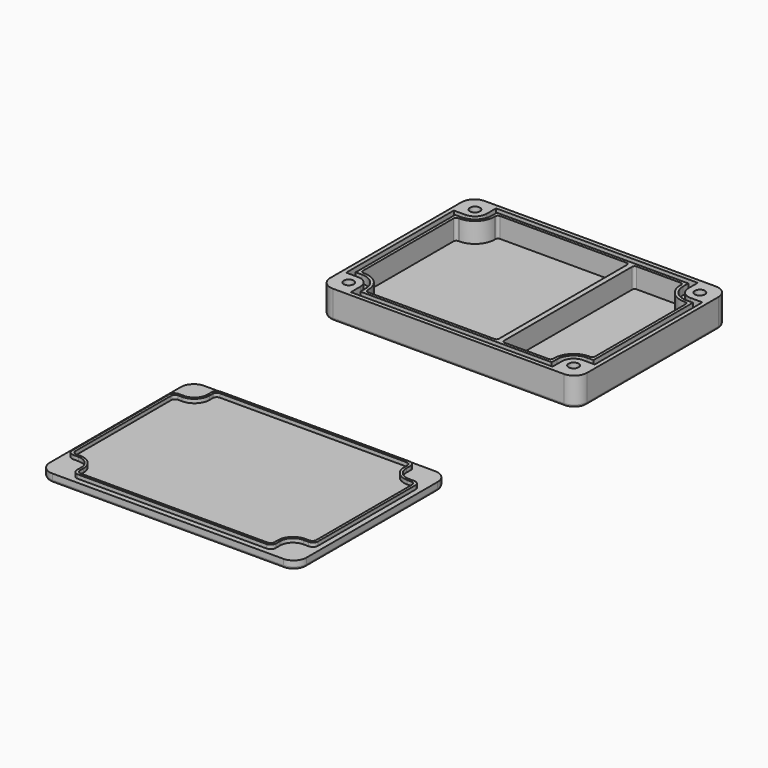
from build123d import *

# Parameters (mm, degrees)
F0_R      = 1.95
F1_DEPTH  = 11
F2_DEPTH  = 8
F3_DEPTH  = 3.2
F4_R      = 1.25
F5_DEPTH  = 3.2
F4_W      = 2
F4_H      = 66.4
F6_DEPTH  = 4.7
F4_R_2    = 2.75
F7_DEPTH  = 3.2
F8_DEPTH  = 3.2
F9_DEPTH  = 3.2
F10_R     = 1
F10_2_R   = 1
F12_R     = 3.65
F12_R_2   = 1.95
F13_DEPTH = 3.7
F17_DEPTH = 1.5
F18_DEPTH = 1.5
F19_R     = 2


# Not quite as in the source:
# - two fillets or chamfers of one size are made in one step


with BuildPart() as f1:
    # F0 (on Top) → F1 (new body)
    with BuildSketch(Plane.XY):
        with BuildLine():
            Line((56.8, 36.8), (-32.8, 36.8))
            ThreePointArc((-32.8, 36.8), (-36.3355339059, 35.3355339059), (-37.8, 31.8))
            Line((-37.8, 31.8), (-37.8, -31.8))
            ThreePointArc((-37.8, -31.8), (-36.3355339059, -35.3355339059), (-32.8, -36.8))
            Line((-32.8, -36.8), (56.8, -36.8))
            ThreePointArc((56.8, -36.8), (60.3355339059, -35.3355339059), (61.8, -31.8))
            Line((61.8, -31.8), (61.8, 31.8))
            ThreePointArc((61.8, 31.8), (60.3355339059, 35.3355339059), (56.8, 36.8))
        make_face()
        with Locations((-31.6, -30.6)):
            Circle(F0_R, mode=Mode.SUBTRACT)
        with Locations((55.6, -30.6)):
            Circle(F0_R, mode=Mode.SUBTRACT)
        with BuildLine():
            Line((51.1, -35.2), (-27.1, -35.2))
            Line((-27.1, -35.2), (-27.1, -30.6))
            ThreePointArc((-27.1, -30.6), (-28.4180194847, -27.4180194847), (-31.6, -26.1))
            Line((-31.6, -26.1), (-36.2, -26.1))
            Line((-36.2, -26.1), (-36.2, 26.1))
            Line((-36.2, 26.1), (-31.6, 26.1))
            ThreePointArc((-31.6, 26.1), (-28.4180194847, 27.4180194847), (-27.1, 30.6))
            Line((-27.1, 30.6), (-27.1, 35.2))
            Line((-27.1, 35.2), (51.1, 35.2))
            Line((51.1, 35.2), (51.1, 30.6))
            ThreePointArc((51.1, 30.6), (52.4180194847, 27.4180194847), (55.6, 26.1))
            Line((55.6, 26.1), (60.2, 26.1))
            Line((60.2, 26.1), (60.2, -26.1))
            Line((60.2, -26.1), (55.6, -26.1))
            ThreePointArc((55.6, -26.1), (52.4180194847, -27.4180194847), (51.1, -30.6))
            Line((51.1, -30.6), (51.1, -35.2))
        make_face(mode=Mode.SUBTRACT)
        with Locations((-31.6, 30.6)):
            Circle(F0_R, mode=Mode.SUBTRACT)
        with Locations((55.6, 30.6)):
            Circle(F0_R, mode=Mode.SUBTRACT)
    extrude(amount=F1_DEPTH)



with BuildPart() as f1b:
    # F0 (on Top) → F1, piece 2 (new body)
    with BuildSketch(Plane.XY):
        with BuildLine():
            Line((49.1, 33.1), (-25.1, 33.1))
            Line((-25.1, 33.1), (-25.1, 30.6))
            ThreePointArc((-25.1, 30.6), (-27.0038059223, 26.0038059223), (-31.6, 24.1))
            Line((-31.6, 24.1), (-34.1, 24.1))
            Line((-34.1, 24.1), (-34.1, -24.1))
            Line((-34.1, -24.1), (-31.6, -24.1))
            ThreePointArc((-31.6, -24.1), (-27.0038059223, -26.0038059223), (-25.1, -30.6))
            Line((-25.1, -30.6), (-25.1, -33.1))
            Line((-25.1, -33.1), (49.1, -33.1))
            Line((49.1, -33.1), (49.1, -30.6))
            ThreePointArc((49.1, -30.6), (51.0038059223, -26.0038059223), (55.6, -24.1))
            Line((55.6, -24.1), (58.1, -24.1))
            Line((58.1, -24.1), (58.1, 24.1))
            Line((58.1, 24.1), (55.6, 24.1))
            ThreePointArc((55.6, 24.1), (51.0038059223, 26.0038059223), (49.1, 30.6))
            Line((49.1, 30.6), (49.1, 33.1))
        make_face()
        with BuildLine():
            Line((-24, 30.6), (-24, 32))
            Line((-24, 32), (27, 32))
            Line((27, 32), (27, -32))
            Line((27, -32), (-24, -32))
            Line((-24, -32), (-24, -30.6))
            ThreePointArc((-24, -30.6), (-26.225988463, -25.225988463), (-31.6, -23))
            Line((-31.6, -23), (-33, -23))
            Line((-33, -23), (-33, 23))
            Line((-33, 23), (-31.6, 23))
            ThreePointArc((-31.6, 23), (-26.225988463, 25.225988463), (-24, 30.6))
        make_face(mode=Mode.SUBTRACT)
        with BuildLine():
            Line((55.6, 23), (57, 23))
            Line((57, 23), (57, -23))
            Line((57, -23), (55.6, -23))
            ThreePointArc((55.6, -23), (50.225988463, -25.225988463), (48, -30.6))
            Line((48, -30.6), (48, -32))
            Line((48, -32), (29, -32))
            Line((29, -32), (29, 32))
            Line((29, 32), (48, 32))
            Line((48, 32), (48, 30.6))
            ThreePointArc((48, 30.6), (50.225988463, 25.225988463), (55.6, 23))
        make_face(mode=Mode.SUBTRACT)
    extrude(amount=F1_DEPTH)


with BuildPart() as f1_1:
    add(f1.part)

    add(f1b.part)  # F2 merges F1b
    # F0 (on Top) → F2 (join)
    with BuildSketch(Plane.XY):
        with BuildLine():
            Line((-27.1, -30.6), (-27.1, -35.2))
            Line((-27.1, -35.2), (51.1, -35.2))
            Line((51.1, -35.2), (51.1, -30.6))
            ThreePointArc((51.1, -30.6), (52.4180194847, -27.4180194847), (55.6, -26.1))
            Line((55.6, -26.1), (60.2, -26.1))
            Line((60.2, -26.1), (60.2, 26.1))
            Line((60.2, 26.1), (55.6, 26.1))
            ThreePointArc((55.6, 26.1), (52.4180194847, 27.4180194847), (51.1, 30.6))
            Line((51.1, 30.6), (51.1, 35.2))
            Line((51.1, 35.2), (-27.1, 35.2))
            Line((-27.1, 35.2), (-27.1, 30.6))
            ThreePointArc((-27.1, 30.6), (-28.4180194847, 27.4180194847), (-31.6, 26.1))
            Line((-31.6, 26.1), (-36.2, 26.1))
            Line((-36.2, 26.1), (-36.2, -26.1))
            Line((-36.2, -26.1), (-31.6, -26.1))
            ThreePointArc((-31.6, -26.1), (-28.4180194847, -27.4180194847), (-27.1, -30.6))
        make_face()
        with BuildLine():
            Line((-25.1, 30.6), (-25.1, 33.1))
            Line((-25.1, 33.1), (49.1, 33.1))
            Line((49.1, 33.1), (49.1, 30.6))
            ThreePointArc((49.1, 30.6), (51.0038059223, 26.0038059223), (55.6, 24.1))
            Line((55.6, 24.1), (58.1, 24.1))
            Line((58.1, 24.1), (58.1, -24.1))
            Line((58.1, -24.1), (55.6, -24.1))
            ThreePointArc((55.6, -24.1), (51.0038059223, -26.0038059223), (49.1, -30.6))
            Line((49.1, -30.6), (49.1, -33.1))
            Line((49.1, -33.1), (-25.1, -33.1))
            Line((-25.1, -33.1), (-25.1, -30.6))
            ThreePointArc((-25.1, -30.6), (-27.0038059223, -26.0038059223), (-31.6, -24.1))
            Line((-31.6, -24.1), (-34.1, -24.1))
            Line((-34.1, -24.1), (-34.1, 24.1))
            Line((-34.1, 24.1), (-31.6, 24.1))
            ThreePointArc((-31.6, 24.1), (-27.0038059223, 26.0038059223), (-25.1, 30.6))
        make_face(mode=Mode.SUBTRACT)
    extrude(amount=F2_DEPTH)

    # F0 (on Top) → F3 (join)
    with BuildSketch(Plane.XY):
        with BuildLine():
            Line((57, -23), (57, 23))
            Line((57, 23), (55.6, 23))
            ThreePointArc((55.6, 23), (50.225988463, 25.225988463), (48, 30.6))
            Line((48, 30.6), (48, 32))
            Line((48, 32), (29, 32))
            Line((29, 32), (29, -32))
            Line((29, -32), (48, -32))
            Line((48, -32), (48, -30.6))
            ThreePointArc((48, -30.6), (50.225988463, -25.225988463), (55.6, -23))
            Line((55.6, -23), (57, -23))
        make_face()
        with BuildLine():
            Line((27, 32), (-24, 32))
            Line((-24, 32), (-24, 30.6))
            ThreePointArc((-24, 30.6), (-26.225988463, 25.225988463), (-31.6, 23))
            Line((-31.6, 23), (-33, 23))
            Line((-33, 23), (-33, -23))
            Line((-33, -23), (-31.6, -23))
            ThreePointArc((-31.6, -23), (-26.225988463, -25.225988463), (-24, -30.6))
            Line((-24, -30.6), (-24, -32))
            Line((-24, -32), (27, -32))
            Line((27, -32), (27, 32))
        make_face()
    extrude(amount=F3_DEPTH)

    # F10#2
    f10_2_edges = [f1_1.edges().sort_by_distance(p)[0] for p in [
        (-24, 32, 7.1),
        (27, 32, 7.1),
        (27, -32, 7.1),
        (-24, -32, 7.1),
        (-33, -23, 7.1),
        (-33, 23, 7.1),
        (57, 23, 7.1),
        (57, -23, 7.1),
        (48, -32, 7.1),
        (29, -32, 7.1),
        (29, 32, 7.1),
        (48, 32, 7.1),
        (12, 36.8, 0),
        (-36.335534, 35.335534, 0),
        (-37.8, 0, 0),
        (-36.335534, -35.335534, 0),
        (12, -36.8, 0),
        (60.335534, -35.335534, 0),
        (61.8, 0, 0),
        (60.335534, 35.335534, 0),
    ]]
    fillet(f10_2_edges, radius=F10_2_R)

    # F12 (on face) → F13 (cut)
    with BuildSketch(Plane(origin=(0, 0, 0), x_dir=(1, 0, 0), z_dir=(0, 0, -1))):
        with Locations((55.6, -30.6)):
            Circle(F12_R)
        with Locations((55.6, -30.6)):
            Circle(F12_R_2, mode=Mode.SUBTRACT)
        with Locations((55.6, 30.6)):
            Circle(F12_R)
        with Locations((55.6, 30.6)):
            Circle(F12_R_2, mode=Mode.SUBTRACT)
        with Locations((-31.6, -30.6)):
            Circle(F12_R)
        with Locations((-31.6, -30.6)):
            Circle(F12_R_2, mode=Mode.SUBTRACT)
        with Locations((-31.6, 30.6)):
            Circle(F12_R)
        with Locations((-31.6, 30.6)):
            Circle(F12_R_2, mode=Mode.SUBTRACT)
    extrude(amount=-F13_DEPTH, mode=Mode.SUBTRACT)


with BuildPart() as f5:
    # F4 (on Top) → F5 (new body)
    with BuildSketch(Plane.XY):
        with BuildLine():
            Line((56.8, -99.2), (-32.8, -99.2))
            ThreePointArc((-32.8, -99.2), (-36.3355339059, -100.6644660941), (-37.8, -104.2))
            Line((-37.8, -104.2), (-37.8, -167.8))
            ThreePointArc((-37.8, -167.8), (-36.3355339059, -171.3355339059), (-32.8, -172.8))
            Line((-32.8, -172.8), (56.8, -172.8))
            ThreePointArc((56.8, -172.8), (60.3355339059, -171.3355339059), (61.8, -167.8))
            Line((61.8, -167.8), (61.8, -104.2))
            ThreePointArc((61.8, -104.2), (60.3355339059, -100.6644660941), (56.8, -99.2))
        make_face()
        with Locations((-31.6, -166.6)):
            Circle(F4_R, mode=Mode.SUBTRACT)
        with Locations((55.6, -166.6)):
            Circle(F4_R, mode=Mode.SUBTRACT)
        with BuildLine():
            Line((-27, -105.4), (-27, -100.9))
            Line((-27, -100.9), (51, -100.9))
            Line((51, -100.9), (51.0491758988, -100.9))
            ThreePointArc((51.0491758988, -100.9), (51.0245188805, -100.9250729028), (51, -100.9502809077))
            Line((51, -100.9502809077), (51, -105.4))
            ThreePointArc((51, -105.4), (52.3473088065, -108.6526911935), (55.6, -110))
            Line((55.6, -110), (60.0497190923, -110))
            ThreePointArc((60.0497190923, -110), (60.0749270972, -109.9754811195), (60.1, -109.9508241012))
            Line((60.1, -109.9508241012), (60.1, -110))
            Line((60.1, -110), (60.1, -162))
            Line((60.1, -162), (60.1, -162.0491758988))
            ThreePointArc((60.1, -162.0491758988), (60.0749270972, -162.0245188805), (60.0497190923, -162))
            Line((60.0497190923, -162), (55.6, -162))
            ThreePointArc((55.6, -162), (52.3473088065, -163.3473088065), (51, -166.6))
            Line((51, -166.6), (51, -171.0497190923))
            ThreePointArc((51, -171.0497190923), (51.0245188805, -171.0749270972), (51.0491758988, -171.1))
            Line((51.0491758988, -171.1), (51, -171.1))
            Line((51, -171.1), (-27, -171.1))
            Line((-27, -171.1), (-27.0491758988, -171.1))
            ThreePointArc((-27.0491758988, -171.1), (-27.0245188805, -171.0749270972), (-27, -171.0497190923))
            Line((-27, -171.0497190923), (-27, -166.6))
            ThreePointArc((-27, -166.6), (-28.3473088065, -163.3473088065), (-31.6, -162))
            Line((-31.6, -162), (-36.0497190923, -162))
            ThreePointArc((-36.0497190923, -162), (-36.0749270972, -162.0245188805), (-36.1, -162.0491758988))
            Line((-36.1, -162.0491758988), (-36.1, -162))
            Line((-36.1, -162), (-36.1, -110))
            Line((-36.1, -110), (-31.6, -110))
            ThreePointArc((-31.6, -110), (-28.3473088065, -108.6526911935), (-27, -105.4))
        make_face(mode=Mode.SUBTRACT)
        with Locations((-31.6, -105.4)):
            Circle(F4_R, mode=Mode.SUBTRACT)
        with Locations((55.6, -105.4)):
            Circle(F4_R, mode=Mode.SUBTRACT)
    extrude(amount=F5_DEPTH)



with BuildPart() as f5b:
    # F4 (on Top) → F5, piece 2 (new body)
    with BuildSketch(Plane.XY):
        with Locations((28, -136)):
            Rectangle(F4_W, F4_H)
    extrude(amount=F5_DEPTH)


with BuildPart() as f5_1:
    add(f5.part)

    add(f5b.part)  # F6 merges F5b
    # F4 (on Top) → F6 (join)
    with BuildSketch(Plane.XY):
        with BuildLine():
            Line((51, -100.9), (-27, -100.9))
            Line((-27, -100.9), (-27, -105.4))
            ThreePointArc((-27, -105.4), (-28.3473088065, -108.6526911935), (-31.6, -110))
            Line((-31.6, -110), (-36.1, -110))
            Line((-36.1, -110), (-36.1, -162))
            Line((-36.1, -162), (-36.0497190923, -162))
            Line((-36.0497190923, -162), (-31.6, -162))
            ThreePointArc((-31.6, -162), (-28.3473088065, -163.3473088065), (-27, -166.6))
            Line((-27, -166.6), (-27, -171.0497190923))
            Line((-27, -171.0497190923), (-27, -171.1))
            Line((-27, -171.1), (51, -171.1))
            Line((51, -171.1), (51, -171.0497190923))
            Line((51, -171.0497190923), (51, -166.6))
            ThreePointArc((51, -166.6), (52.3473088065, -163.3473088065), (55.6, -162))
            Line((55.6, -162), (60.0497190923, -162))
            Line((60.0497190923, -162), (60.1, -162))
            Line((60.1, -162), (60.1, -110))
            Line((60.1, -110), (60.0497190923, -110))
            Line((60.0497190923, -110), (55.6, -110))
            ThreePointArc((55.6, -110), (52.3473088065, -108.6526911935), (51, -105.4))
            Line((51, -105.4), (51, -100.9502809077))
            Line((51, -100.9502809077), (51, -100.9))
        make_face()
        with BuildLine():
            Line((-25.2, -105.4), (-25.2, -102.8))
            Line((-25.2, -102.8), (27, -102.8))
            Line((27, -102.8), (29, -102.8))
            Line((29, -102.8), (49.2, -102.8))
            Line((49.2, -102.8), (49.2, -105.4))
            ThreePointArc((49.2, -105.4), (51.0745166004, -109.9254833996), (55.6, -111.8))
            Line((55.6, -111.8), (58.2, -111.8))
            Line((58.2, -111.8), (58.2, -160.2))
            Line((58.2, -160.2), (55.6, -160.2))
            ThreePointArc((55.6, -160.2), (51.0745166004, -162.0745166004), (49.2, -166.6))
            Line((49.2, -166.6), (49.2, -169.2))
            Line((49.2, -169.2), (29, -169.2))
            Line((29, -169.2), (27, -169.2))
            Line((27, -169.2), (-25.2, -169.2))
            Line((-25.2, -169.2), (-25.2, -166.6))
            ThreePointArc((-25.2, -166.6), (-27.0745166004, -162.0745166004), (-31.6, -160.2))
            Line((-31.6, -160.2), (-34.2, -160.2))
            Line((-34.2, -160.2), (-34.2, -111.8))
            Line((-34.2, -111.8), (-31.6, -111.8))
            ThreePointArc((-31.6, -111.8), (-27.0745166004, -109.9254833996), (-25.2, -105.4))
        make_face(mode=Mode.SUBTRACT)
    extrude(amount=F6_DEPTH)

    # F4 (on Top) → F7 (join)
    with BuildSketch(Plane.XY):
        with Locations((-31.6, -105.4)):
            Circle(F4_R)
        with Locations((55.6, -105.4)):
            Circle(F4_R)
        with Locations((-31.6, -166.6)):
            Circle(F4_R)
        with Locations((55.6, -166.6)):
            Circle(F4_R)
        with BuildLine():
            Line((49.2, -102.8), (29, -102.8))
            Line((29, -102.8), (29, -169.2))
            Line((29, -169.2), (49.2, -169.2))
            Line((49.2, -169.2), (49.2, -166.6))
            ThreePointArc((49.2, -166.6), (51.0745166004, -162.0745166004), (55.6, -160.2))
            Line((55.6, -160.2), (58.2, -160.2))
            Line((58.2, -160.2), (58.2, -111.8))
            Line((58.2, -111.8), (55.6, -111.8))
            ThreePointArc((55.6, -111.8), (51.0745166004, -109.9254833996), (49.2, -105.4))
            Line((49.2, -105.4), (49.2, -102.8))
        make_face()
        with BuildLine():
            Line((27, -102.8), (-25.2, -102.8))
            Line((-25.2, -102.8), (-25.2, -105.4))
            ThreePointArc((-25.2, -105.4), (-27.0745166004, -109.9254833996), (-31.6, -111.8))
            Line((-31.6, -111.8), (-34.2, -111.8))
            Line((-34.2, -111.8), (-34.2, -160.2))
            Line((-34.2, -160.2), (-31.6, -160.2))
            ThreePointArc((-31.6, -160.2), (-27.0745166004, -162.0745166004), (-25.2, -166.6))
            Line((-25.2, -166.6), (-25.2, -169.2))
            Line((-25.2, -169.2), (27, -169.2))
            Line((27, -169.2), (27, -102.8))
        make_face()
        with Locations((-20, -156)):
            Circle(F4_R_2, mode=Mode.SUBTRACT)
        with Locations((20, -156)):
            Circle(F4_R_2, mode=Mode.SUBTRACT)
        with Locations((-20, -116)):
            Circle(F4_R_2, mode=Mode.SUBTRACT)
        with Locations((20, -116)):
            Circle(F4_R_2, mode=Mode.SUBTRACT)
    extrude(amount=F7_DEPTH)

    # F4 (on Top) → F8 (join, through all)
    with BuildSketch(Plane.XY):
        with Locations((-20, -116)):
            Circle(F4_R_2)
        with Locations((-20, -116)):
            Circle(F4_R, mode=Mode.SUBTRACT)
        with Locations((-20, -156)):
            Circle(F4_R_2)
        with Locations((-20, -156)):
            Circle(F4_R, mode=Mode.SUBTRACT)
        with Locations((20, -156)):
            Circle(F4_R_2)
        with Locations((20, -156)):
            Circle(F4_R, mode=Mode.SUBTRACT)
        with Locations((20, -116)):
            Circle(F4_R_2)
        with Locations((20, -116)):
            Circle(F4_R, mode=Mode.SUBTRACT)
    extrude(amount=F8_DEPTH)

    # F4 (on Top) → F9 (join, through all)
    with BuildSketch(Plane.XY):
        with Locations((-20, -116)):
            Circle(F4_R)
        with Locations((20, -116)):
            Circle(F4_R)
        with Locations((20, -156)):
            Circle(F4_R)
        with Locations((-20, -156)):
            Circle(F4_R)
    extrude(amount=F9_DEPTH)

    # F10
    f10_edges = [f5_1.edges().sort_by_distance(p)[0] for p in [
        (49.2, -102.8, 3.95),
        (58.2, -111.8, 3.95),
        (58.2, -160.2, 3.95),
        (49.2, -169.2, 3.95),
        (-25.2, -102.8, 3.95),
        (-34.2, -111.8, 3.95),
        (-25.2, -169.2, 3.95),
        (-34.2, -160.2, 3.95),
        (61.8, -136, 0),
        (60.335534, -171.335534, 0),
        (60.335534, -100.664466, 0),
        (12, -99.2, 0),
        (-36.335534, -100.664466, 0),
        (-37.8, -136, 0),
        (-36.335534, -171.335534, 0),
        (12, -172.8, 0),
    ]]
    fillet(f10_edges, radius=F10_R)

    # F16 (on face) → F17 (cut, through all)
    with BuildSketch(Plane.XY.offset(4.7)):
        with BuildLine():
            Line((-36.1, -110), (-36.1, -162))
            Line((-36.1, -162), (-31.6, -162))
            ThreePointArc((-31.6, -162), (-28.3473088065, -163.3473088065), (-27, -166.6))
            Line((-27, -166.6), (-27, -171.1))
            Line((-27, -171.1), (51, -171.1))
            Line((51, -171.1), (51, -166.6))
            ThreePointArc((51, -166.6), (52.3473088065, -163.3473088065), (55.6, -162))
            Line((55.6, -162), (60.1, -162))
            Line((60.1, -162), (60.1, -110))
            Line((60.1, -110), (55.6, -110))
            ThreePointArc((55.6, -110), (52.3473088065, -108.6526911935), (51, -105.4))
            Line((51, -105.4), (51, -100.9))
            Line((51, -100.9), (-27, -100.9))
            Line((-27, -100.9), (-27, -105.4))
            ThreePointArc((-27, -105.4), (-28.3473088065, -108.6526911935), (-31.6, -110))
            Line((-31.6, -110), (-36.1, -110))
        make_face()
        with BuildLine():
            ThreePointArc((-31.6, -110.4), (-28.0644660941, -108.9355339059), (-26.6, -105.4))
            Line((-26.6, -105.4), (-26.6, -101.3))
            Line((-26.6, -101.3), (50.6, -101.3))
            Line((50.6, -101.3), (50.6, -105.4))
            ThreePointArc((50.6, -105.4), (52.0644660941, -108.9355339059), (55.6, -110.4))
            Line((55.6, -110.4), (59.7, -110.4))
            Line((59.7, -110.4), (59.7, -161.6))
            Line((59.7, -161.6), (55.6, -161.6))
            ThreePointArc((55.6, -161.6), (52.0644660941, -163.0644660941), (50.6, -166.6))
            Line((50.6, -166.6), (50.6, -170.7))
            Line((50.6, -170.7), (-26.6, -170.7))
            Line((-26.6, -170.7), (-26.6, -166.6))
            ThreePointArc((-26.6, -166.6), (-28.0644660941, -163.0644660941), (-31.6, -161.6))
            Line((-31.6, -161.6), (-35.7, -161.6))
            Line((-35.7, -161.6), (-35.7, -110.4))
            Line((-35.7, -110.4), (-31.6, -110.4))
        make_face(mode=Mode.SUBTRACT)
    extrude(amount=-F17_DEPTH, mode=Mode.SUBTRACT)

    # F16 (on face) → F18 (cut, through all)
    with BuildSketch(Plane.XY.offset(4.7)):
        with BuildLine():
            ThreePointArc((58.7, -112.8), (58.2606601718, -111.7393398282), (57.2, -111.3))
            Line((57.2, -111.3), (55.6, -111.3))
            ThreePointArc((55.6, -111.3), (51.428069991, -109.571930009), (49.7, -105.4))
            Line((49.7, -105.4), (49.7, -103.8))
            ThreePointArc((49.7, -103.8), (49.2606601718, -102.7393398282), (48.2, -102.3))
            Line((48.2, -102.3), (-24.2, -102.3))
            ThreePointArc((-24.2, -102.3), (-25.2606601718, -102.7393398282), (-25.7, -103.8))
            Line((-25.7, -103.8), (-25.7, -105.4))
            ThreePointArc((-25.7, -105.4), (-27.428069991, -109.571930009), (-31.6, -111.3))
            Line((-31.6, -111.3), (-33.2, -111.3))
            ThreePointArc((-33.2, -111.3), (-34.2606601718, -111.7393398282), (-34.7, -112.8))
            Line((-34.7, -112.8), (-34.7, -159.2))
            ThreePointArc((-34.7, -159.2), (-34.2606601718, -160.2606601718), (-33.2, -160.7))
            Line((-33.2, -160.7), (-31.6, -160.7))
            ThreePointArc((-31.6, -160.7), (-27.428069991, -162.428069991), (-25.7, -166.6))
            Line((-25.7, -166.6), (-25.7, -168.2))
            ThreePointArc((-25.7, -168.2), (-25.2606601718, -169.2606601718), (-24.2, -169.7))
            Line((-24.2, -169.7), (48.2, -169.7))
            ThreePointArc((48.2, -169.7), (49.2606601718, -169.2606601718), (49.7, -168.2))
            Line((49.7, -168.2), (49.7, -166.6))
            ThreePointArc((49.7, -166.6), (51.428069991, -162.428069991), (55.6, -160.7))
            Line((55.6, -160.7), (57.2, -160.7))
            ThreePointArc((57.2, -160.7), (58.2606601718, -160.2606601718), (58.7, -159.2))
            Line((58.7, -159.2), (58.7, -112.8))
        make_face()
        with BuildLine():
            ThreePointArc((-25.2, -103.8), (-24.9071067812, -103.0928932188), (-24.2, -102.8))
            Line((-24.2, -102.8), (48.2, -102.8))
            ThreePointArc((48.2, -102.8), (48.9071067812, -103.0928932188), (49.2, -103.8))
            Line((49.2, -103.8), (49.2, -105.4))
            ThreePointArc((49.2, -105.4), (51.0745166004, -109.9254833996), (55.6, -111.8))
            Line((55.6, -111.8), (57.2, -111.8))
            ThreePointArc((57.2, -111.8), (57.9071067812, -112.0928932188), (58.2, -112.8))
            Line((58.2, -112.8), (58.2, -159.2))
            ThreePointArc((58.2, -159.2), (57.9071067812, -159.9071067812), (57.2, -160.2))
            Line((57.2, -160.2), (55.6, -160.2))
            ThreePointArc((55.6, -160.2), (51.0745166004, -162.0745166004), (49.2, -166.6))
            Line((49.2, -166.6), (49.2, -168.2))
            ThreePointArc((49.2, -168.2), (48.9071067812, -168.9071067812), (48.2, -169.2))
            Line((48.2, -169.2), (-24.2, -169.2))
            ThreePointArc((-24.2, -169.2), (-24.9071067812, -168.9071067812), (-25.2, -168.2))
            Line((-25.2, -168.2), (-25.2, -166.6))
            ThreePointArc((-25.2, -166.6), (-27.0745166004, -162.0745166004), (-31.6, -160.2))
            Line((-31.6, -160.2), (-33.2, -160.2))
            ThreePointArc((-33.2, -160.2), (-33.9071067812, -159.9071067812), (-34.2, -159.2))
            Line((-34.2, -159.2), (-34.2, -112.8))
            ThreePointArc((-34.2, -112.8), (-33.9071067812, -112.0928932188), (-33.2, -111.8))
            Line((-33.2, -111.8), (-31.6, -111.8))
            ThreePointArc((-31.6, -111.8), (-27.0745166004, -109.9254833996), (-25.2, -105.4))
            Line((-25.2, -105.4), (-25.2, -103.8))
        make_face(mode=Mode.SUBTRACT)
    extrude(amount=-F18_DEPTH, mode=Mode.SUBTRACT)

    # F19
    f19_edges = [f5_1.edges().sort_by_distance(p)[0] for p in [
        (59.7, -161.6, 3.95),
        (50.6, -170.7, 3.95),
        (-26.6, -170.7, 3.95),
        (-35.7, -161.6, 3.95),
        (-35.7, -110.4, 3.95),
        (-26.6, -101.3, 3.95),
        (50.6, -101.3, 3.95),
        (59.7, -110.4, 3.95),
    ]]
    fillet(f19_edges, radius=F19_R)


solid = Compound([f1_1.part, f5_1.part])
